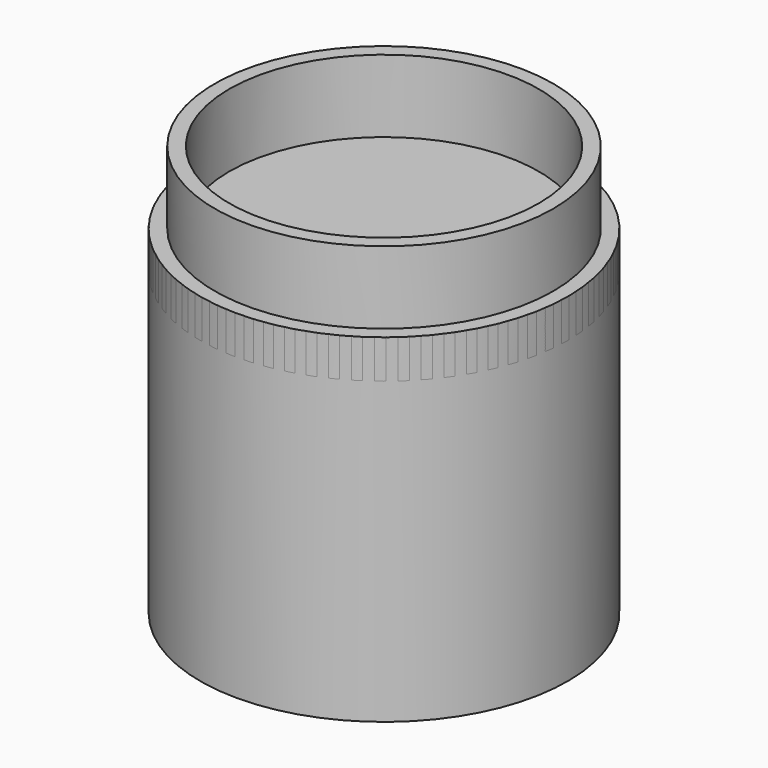
from build123d import *

# Parameters (mm, degrees)
F1_DEPTH = 88.9
F2_R     = 48.26
F2_R_2   = 30.48
F3_DEPTH = 10.16
F4_R     = 44.45
F4_R_2   = 40.64
F5_DEPTH = 19.05
F6_DEPTH = 5.08


# Not quite as in the source:
# - a feature names something its author has since deleted; it is built from what else it names


with BuildPart() as f1:
    # F0 (on Top) → F1 (new body)
    with BuildSketch(Plane.XY):
        with BuildLine():
            ThreePointArc((-12.7063658778, 46.5572321576), (0, -48.26), (12.7063658778, 46.5572321576))
            Line((12.7063658778, 46.5572321576), (12.7063658778, 42.5951579627))
            ThreePointArc((12.7063658778, 42.5951579627), (0, -44.4500385526), (-12.7063658778, 42.5951579627))
            Line((-12.7063658778, 42.5951579627), (-12.7063658778, 46.5572321576))
        make_face()
    extrude(amount=-F1_DEPTH)


with BuildPart() as f3:
    # F2 (on Top) → F3 (new body)
    with BuildSketch(Plane.XY):
        Circle(F2_R)
        Circle(F2_R_2, mode=Mode.SUBTRACT)
        Circle(F2_R_2)
    extrude(amount=-F3_DEPTH)


with BuildPart() as f5:
    # F4 (on Top) → F5 (new body)
    with BuildSketch(Plane.XY):
        Circle(F4_R)
        Circle(F4_R_2, mode=Mode.SUBTRACT)
    extrude(amount=F5_DEPTH)


with BuildPart() as f6:
    # F4 (on Top) → F6 (new body)
    with BuildSketch(Plane.XY):
        Circle(F4_R)
        Circle(F4_R_2, mode=Mode.SUBTRACT)
    extrude(amount=-F6_DEPTH)


solid = Compound([f1.part, f3.part, f5.part, f6.part])
